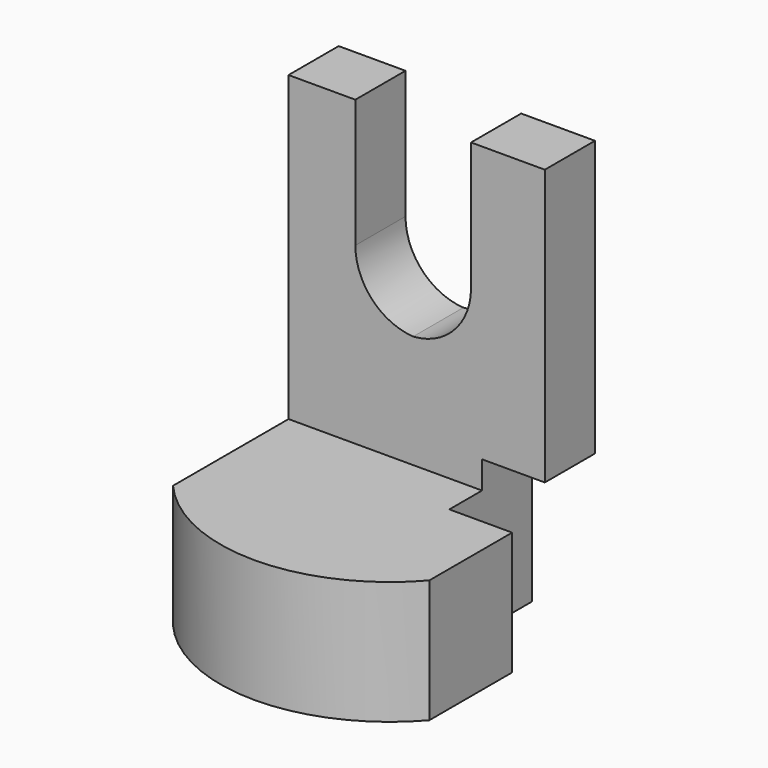
from build123d import *

# Parameters (mm, degrees)
F1_DEPTH    = 25.4
F2_W        = 52.878184244
F2_H        = 12.9309091717
F3_DEPTH    = 87.884
F4_W        = 23.8667652011
F4_H        = 39.1564019587
F5_DEPTH    = 25.4
F6_T1_DEPTH = 12.9309091717
F8_DEPTH    = 12.954


# Not quite as in the source:
# - a fillet or chamfer that OpenCascade refuses, or shapes differently, is made with other operations: its cross-section is extruded or revolved along the edge and cut away or added


with BuildPart() as f1:
    # F0 (on Top) → F1 (new body)
    with BuildSketch(Plane.XY):
        with BuildLine():
            Line((25.1690931618, 17.8954545408), (-27.7090910822, 17.8954545408))
            Line((-27.7090910822, 17.8954545408), (-27.7090910822, -11.891817674))
            ThreePointArc((-27.7090910822, -11.891817674), (-1.2699989602, -23.9832848769), (25.1690931618, -11.891817674))
            Line((25.1690931618, -11.891817674), (25.1690931618, 17.8954545408))
        make_face()
    extrude(amount=F1_DEPTH)

    # F2 (on face) → F3 (join)
    with BuildSketch(Plane(origin=(0, 0, 0), x_dir=(1, 0, 0), z_dir=(0, 0, -1))):
        with Locations((-1.2699989602, -24.3609091267)):
            Rectangle(F2_W, F2_H)
    extrude(amount=-F3_DEPTH)

    # F4 (on face) → F5 (cut)
    with BuildSketch(Plane.XZ.offset(-17.8954545408)):
        with Locations((-1.9888961688, 68.3057990206)):
            Rectangle(F4_W, F4_H)
    extrude(amount=-F5_DEPTH, mode=Mode.SUBTRACT)

    # F6: fillet of radius 12.7 on 2 edges, made by hand

    # F6_s2 → F6_t1 (join)
    with BuildSketch(Plane.XZ.offset(-30.8263637125)):
        with BuildLine():
            ThreePointArc((-13.9222787693, 61.4275980413), (-10.2025348904, 52.4473419202), (-1.2222787693, 48.7275980413))
            Line((-1.2222787693, 48.7275980413), (-13.9222787693, 48.7275980413))
            Line((-13.9222787693, 48.7275980413), (-13.9222787693, 61.4275980413))
        make_face()
        with BuildLine():
            ThreePointArc((-2.7555135682, 48.7275980413), (6.2247425528, 52.4473419202), (9.9444864318, 61.4275980413))
            Line((9.9444864318, 61.4275980413), (9.9444864318, 48.7275980413))
            Line((9.9444864318, 48.7275980413), (-2.7555135682, 48.7275980413))
        make_face()
    extrude(amount=F6_T1_DEPTH)

    # F7 (on face) → F8 (cut)
    with BuildSketch(Plane.YZ.offset(25.1690931618)):
        Polygon((30.8263637125, 0), (30.8263637125, 31.0761313885), (17.8954545408, 31.0761313885), (17.8954545408, 25.4), (9.4672730193, 25.4), (9.4672730193, 0), align=None)
    extrude(amount=-F8_DEPTH, mode=Mode.SUBTRACT)


solid = f1.part
